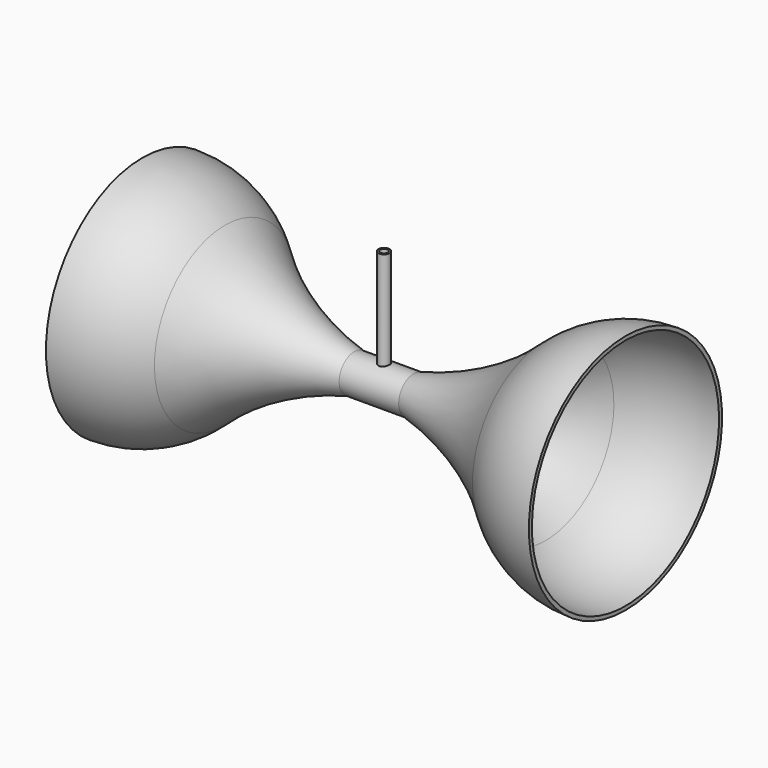
from build123d import *

# Parameters (mm, degrees)
F7_R     = 1.5875
F8_DEPTH = 44.45


# Not quite as in the source:
# - a length typed as a fraction of an inch, garbled in the dataset ("3 / 203.2 mm" for 3/8 in), is restored
# - a feature names something its author has since deleted; it is built from what else it names


with BuildPart() as f5:
    # F4 (on Front) → F5 (revolve)
    with BuildSketch(Plane.XZ):
        with BuildLine():
            ThreePointArc((-57.8191946572, 81.1773013498), (-32.1183318105, 62.7606186977), (-2.5394843148, 51.5892118125))
            Line((-2.5394843148, 51.5892118125), (7.7792656852, 51.5892118125))
            Line((7.7792656852, 51.5892118125), (7.7792656852, 53.1767118125))
            Line((7.7792656852, 53.1767118125), (-2.3548589537, 53.1767118125))
            ThreePointArc((-2.3548589537, 53.1767118125), (-31.4500310941, 64.2035504476), (-56.7346691844, 82.3365945607))
            ThreePointArc((-56.7346691844, 82.3365945607), (-72.7834805037, 92.4895400844), (-91.4394843148, 96.0392118125))
            Line((-91.4394843148, 96.0392118125), (-91.4394843148, 94.4517118125))
            ThreePointArc((-91.4394843148, 94.4517118125), (-73.3664806228, 91.0129673259), (-57.8191946572, 81.1773013498))
        make_face()
        with BuildLine():
            Line((10.1605156852, 53.1767118125), (10.1605156852, 51.5892118125))
            Line((10.1605156852, 51.5892118125), (22.8605156852, 51.5892118125))
            ThreePointArc((22.8605156852, 51.5892118125), (52.439363181, 62.7606186977), (78.1402260277, 81.1773013498))
            ThreePointArc((78.1402260277, 81.1773013498), (93.6875119933, 91.0129673259), (111.7605156852, 94.4517118125))
            Line((111.7605156852, 94.4517118125), (111.7605156852, 96.0392118125))
            ThreePointArc((111.7605156852, 96.0392118125), (93.1045118742, 92.4895400844), (77.0557005549, 82.3365945607))
            ThreePointArc((77.0557005549, 82.3365945607), (51.7710624646, 64.2035504476), (22.6758903242, 53.1767118125))
            Line((22.6758903242, 53.1767118125), (10.3451410463, 53.1767118125))
            Line((10.3451410463, 53.1767118125), (10.1605156852, 53.1767118125))
        make_face()
        Polygon((7.7792656852, 53.1767118125), (7.7792656852, 51.5892118125), (10.1605156852, 51.5892118125), (10.1605156852, 53.1767118125), (9.9758903242, 53.1767118125), align=None)
    revolve(axis=Axis((-40.6394843148, 0, 45.2392118125), (1, 0, 0)))

    # F4 (on Front) → F6 (revolve)
    with BuildSketch(Plane.XZ):
        Polygon((7.7792656852, 94.4517118125), (7.7792656852, 53.1767118125), (9.9758903242, 53.1767118125), (10.1605156852, 53.1767118125), (10.1605156852, 94.4517118125), align=None)
        Polygon((7.7792656852, 53.1767118125), (7.7792656852, 51.5892118125), (10.1605156852, 51.5892118125), (10.1605156852, 53.1767118125), (9.9758903242, 53.1767118125), align=None)
    revolve(axis=Axis((10.1605156852, 0, 73.0204618125), (0, 0, -1)))

    # F7 (on face) → F8 (cut)
    with BuildSketch(Plane.XY.offset(94.4517118125)):
        with Locations((10.1605156852, 0)):
            Circle(F7_R)
    extrude(amount=-F8_DEPTH, mode=Mode.SUBTRACT)


solid = f5.part
